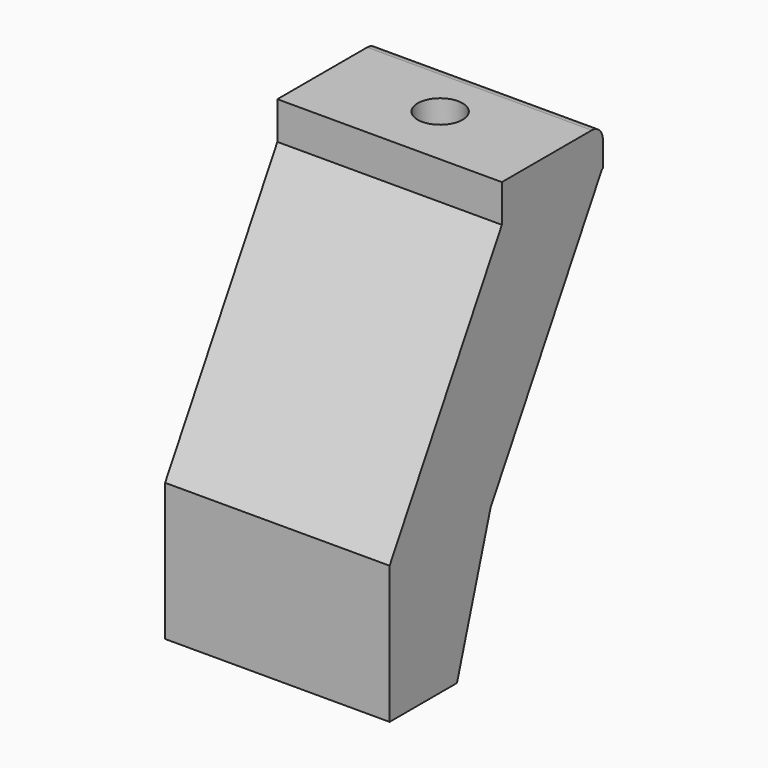
from build123d import *

# Parameters (mm, degrees)
F0_W      = 45
F0_H      = 49
F1_DEPTH  = 80
F3_DEPTH  = 35
F4_W      = 72
F4_H      = 41
F5_DEPTH  = 55
F6_W      = 72
F6_H      = 23
F7_DEPTH  = 15
F9_W      = 80
F9_H      = 45
F9_R      = 8
F10_DEPTH = 14
F11_R     = 5
F13_DEPTH = 80


with BuildPart() as f1:
    # F0 (on Right) → F1 (new body)
    with BuildSketch(Plane.YZ):
        with Locations((22.5, -24.5)):
            Rectangle(F0_W, F0_H)
        Polygon((50, 86.6025403784), (0, 0), (45, 0), (95, 86.6025403784), align=None)
    extrude(amount=F1_DEPTH)

    # F2 (on face) → F3 (cut)
    with BuildSketch(Plane(origin=(0, 33.75, -19.4855715851), x_dir=(-1, 0, 0), z_dir=(0, 0.8660254038, -0.5))):
        Polygon((-76, 22.5), (-4, 22.5), (-4, 117.5), (-4, 122.5), (-76, 122.5), (-76, 117.5), align=None)
    extrude(amount=-F3_DEPTH, mode=Mode.SUBTRACT)

    # F4 (on face) → F5 (cut)
    with BuildSketch(Plane(origin=(0, 0, -49), x_dir=(1, 0, 0), z_dir=(0, 0, -1))):
        with Locations((40, -24.5)):
            Rectangle(F4_W, F4_H)
    extrude(amount=-F5_DEPTH, mode=Mode.SUBTRACT)

    # F6 (on face) → F7 (cut)
    with BuildSketch(Plane(origin=(0, 11.25, 19.4855715851), x_dir=(1, 0, 0), z_dir=(0, 0.5, 0.8660254038))):
        with Locations((40, 15.4711431703)):
            Rectangle(F6_W, F6_H)
    extrude(amount=-F7_DEPTH, mode=Mode.SUBTRACT)

    # F9 (on offset) → F10 (join)
    with BuildSketch(Plane.XY.offset(100)):
        with Locations((40, 72.5)):
            Rectangle(F9_W, F9_H)
        with Locations((40, 72.5)):
            Circle(F9_R, mode=Mode.SUBTRACT)
    extrude(amount=-F10_DEPTH)

    # F11
    f11_edges = [f1.edges().sort_by_distance(p)[0] for p in [
        (40, 95, 100),
    ]]
    fillet(f11_edges, radius=F11_R)

    # F12 (on face) → F13 (cut)
    with BuildSketch(Plane(origin=(0, 0, 0), x_dir=(0, -1, 0), z_dir=(-1, 0, 0))):
        Polygon((-30, -49), (-45, 0), (-45, -49), align=None)
    extrude(amount=-F13_DEPTH, mode=Mode.SUBTRACT)


solid = f1.part
